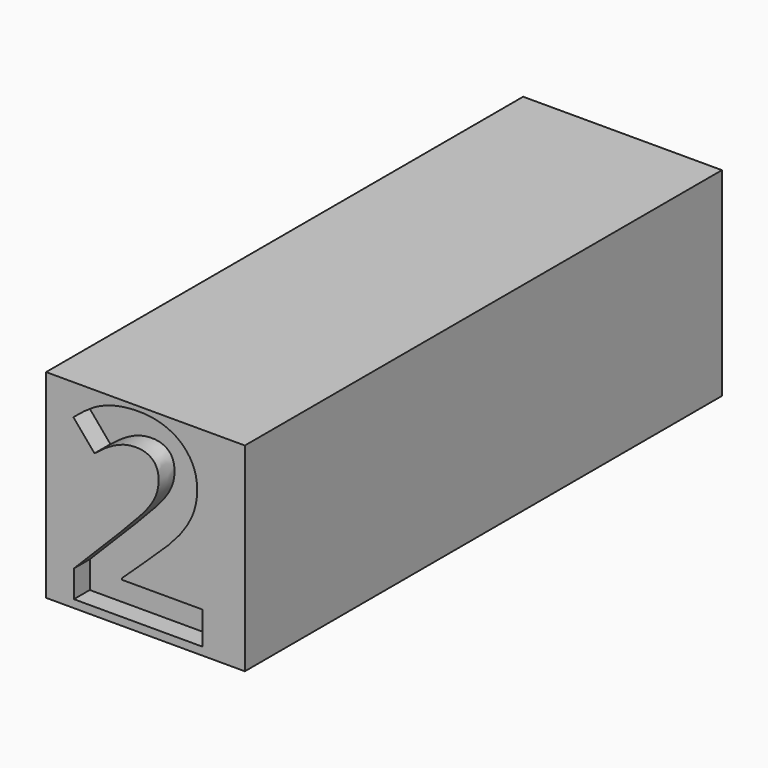
from build123d import *

# Parameters (mm, degrees)
F0_W         = 25.4
F0_H         = 25.4
F1_DEPTH     = 76.2
F2_TEXT_SIZE = 32.8928085057
F3_DEPTH     = 2.54


# Not quite as in the source:
# - Text() gives the source's letters only with a copy of the font that has no kerning and outlines rounded to 1/6400 em; it was checked with that copy


with BuildPart() as f1:
    # F0 (on Front) → F1 (new body)
    with BuildSketch(Plane.XZ):
        with Locations((12.7, 12.7)):
            Rectangle(F0_W, F0_H)
    extrude(amount=F1_DEPTH)

    # F2 (on face) → F3 (cut)
    with BuildSketch(Plane.XZ.offset(76.2)):
        with Locations((2.2344356403, 1.0064573726)):
            Text('2', F2_TEXT_SIZE, font='Open Sans', font_style=FontStyle.BOLD, text_align=(TextAlign.LEFT, TextAlign.BOTTOM))
    extrude(amount=-F3_DEPTH, mode=Mode.SUBTRACT)


solid = f1.part
